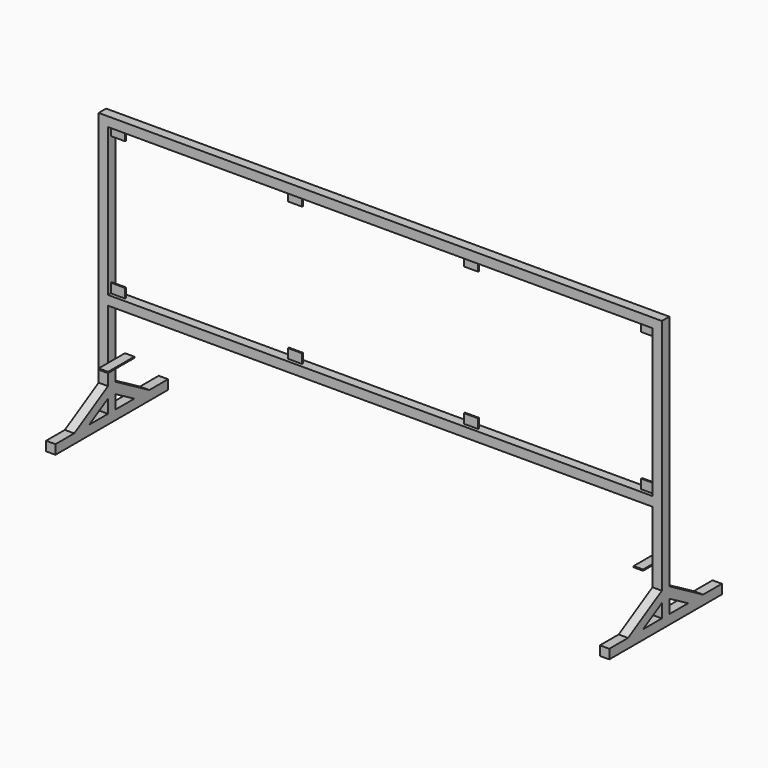
from build123d import *

# Parameters (mm, degrees)
F0_W      = 2320
F0_H      = 630
F0_W_2    = 40
F0_H_2    = 446
F1_DEPTH  = 40
F2_W      = 40
F2_H      = 40
F3_DEPTH  = 40
F4_W      = 50
F4_H      = 5
F4_W_2    = 40
F5_DEPTH  = 40
F9_W      = 60
F9_H      = 40
F10_DEPTH = 5


# Not quite as in the source:
# - a feature names something its author has since deleted; it is built from what else it names


with BuildPart() as f1:
    # F0 (on Front) → F1 (new body)
    with BuildSketch(Plane.XZ):
        Polygon((1200, 432.3376794357), (-1200, 432.3376794357), (-1200, -277.6623205643), (-1160, -277.6623205643), (1160, -277.6623205643), (1200, -277.6623205643), align=None)
        with Locations((0, 77.3376794357)):
            Rectangle(F0_W, F0_H, mode=Mode.SUBTRACT)
        with Locations((1180, -500.6623205643)):
            Rectangle(F0_W_2, F0_H_2)
        with Locations((-1180, -500.6623205643)):
            Rectangle(F0_W_2, F0_H_2)
    extrude(amount=F1_DEPTH)

    # F2 (on face) → F3 (join)
    with BuildSketch(Plane(origin=(-1200, 0, 0), x_dir=(0, -1, 0), z_dir=(-1, 0, 0))):
        Polygon((40, -625.9272936454), (140, -683.6623205643), (220, -683.6623205643), (40, -579.7392721102), align=None)
        Polygon((0, -579.7392721102), (-180, -683.6623205643), (-100, -683.6623205643), (0, -625.9272936454), align=None)
        Polygon((-280, -683.6623205643), (-280, -723.6623205643), (0, -723.6623205643), (0, -683.6623205643), (-100, -683.6623205643), (-180, -683.6623205643), align=None)
        Polygon((40, -683.6623205643), (40, -723.6623205643), (320, -723.6623205643), (320, -683.6623205643), (220, -683.6623205643), (140, -683.6623205643), align=None)
        with Locations((20, -703.6623205643)):
            Rectangle(F2_W, F2_H)
    extrude(amount=-F3_DEPTH)

    # F4 (on face) → F5 (join)
    with BuildSketch(Plane.YZ.offset(-1160)):
        with Locations((25, -495.1623205643)):
            Rectangle(F4_W, F4_H)
        with Locations((-20, -495.1623205643)):
            Rectangle(F4_W_2, F4_H)
        with Locations((-65, -495.1623205643)):
            Rectangle(F4_W, F4_H)
    extrude(amount=F5_DEPTH)

    # F6: F1 across plane


with BuildPart() as f1_1:
    add(f1.part)
    add(f1.part.mirror(Plane.YZ))

    # F7: F1 across plane


with BuildPart() as f1_2:
    add(f1_1.part)
    add(f1_1.part.mirror(Plane.YZ))

    # F9 (on offset) → F10 (join)
    with BuildSketch(Plane.XZ.offset(20)):
        with Locations((-1130, -217.6623205643)):
            Rectangle(F9_W, F9_H)
        with Locations((-1130, 372.3376794357)):
            Rectangle(F9_W, F9_H)
        with Locations((-375, 372.3376794357)):
            Rectangle(F9_W, F9_H)
        with Locations((-375, -217.6623205643)):
            Rectangle(F9_W, F9_H)
        with Locations((375, -217.6623205643)):
            Rectangle(F9_W, F9_H)
        with Locations((375, 372.3376794357)):
            Rectangle(F9_W, F9_H)
        with Locations((1130, 372.3376794357)):
            Rectangle(F9_W, F9_H)
        with Locations((1130, -217.6623205643)):
            Rectangle(F9_W, F9_H)
    extrude(amount=F10_DEPTH)


solid = f1_2.part
